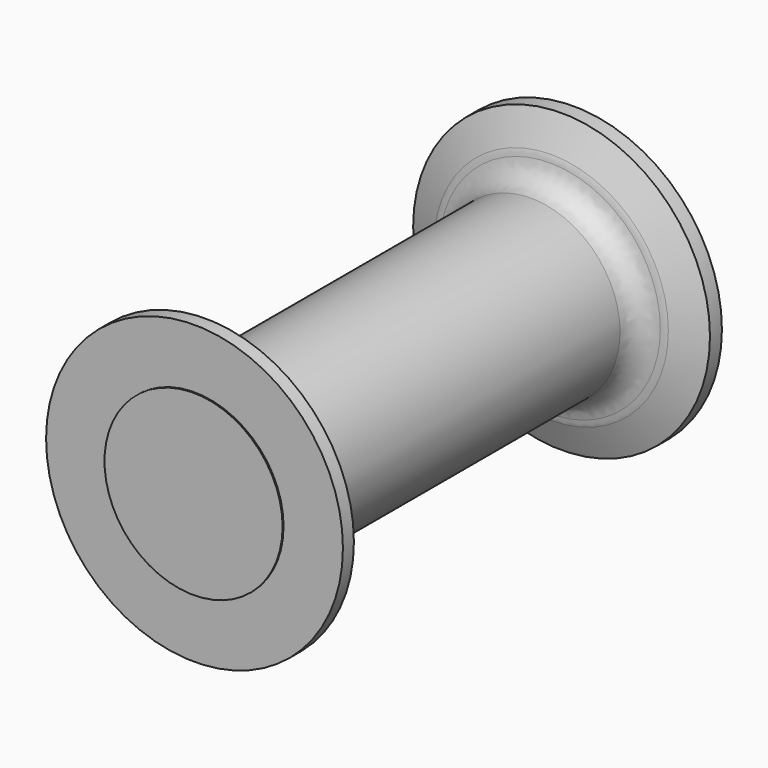
from build123d import *

# Parameters (mm, degrees)
F0_R     = 19.05
F1_DEPTH = 101.6
F2_R     = 31.75
F3_DEPTH = 6.35
F5_START = 95.25
F4_R     = 31.75
F5_DEPTH = 6.096
F6_SIZE  = 2.54
F8_R     = 5.08
F9_R     = 5.08


# Not quite as in the source:
# - a fillet or chamfer that OpenCascade refuses, or shapes differently, is made with other operations: its cross-section is extruded or revolved along the edge and cut away or added


with BuildPart() as f1:
    # F0 (on Front) → F1 (new body)
    with BuildSketch(Plane.XZ):
        Circle(F0_R)
    extrude(amount=F1_DEPTH)

    # F2 (on Front) → F3 (join)
    with BuildSketch(Plane.XZ):
        Circle(F2_R)
    extrude(amount=F3_DEPTH)

    # F4 (on Front) → F5 (join)
    with BuildSketch(Plane.XZ.offset(F5_START)):
        Circle(F4_R)
    extrude(amount=F5_DEPTH)

    # F6
    f6_edges = [f1.edges().sort_by_distance(p)[0] for p in [
        (-31.75, -6.35, 0),
        (-31.75, -95.25, 0),
    ]]
    chamfer(f6_edges, length=F6_SIZE)

    # F7: chamfer of 5.08 on 2 edges, made by hand

    # F7_s1 → F7_t2 (revolve, cut)
    with BuildSketch(Plane.XY):
        Polygon((24.13, -95.25), (32.8021024484, -98.8421024484), (29.21, -95.25), align=None)
    revolve(axis=Axis((0, -95.25, 0), (0, -1, 0)), mode=Mode.SUBTRACT)

    # F7_s3 → F7_t4 (revolve, cut)
    with BuildSketch(Plane.XY):
        Polygon((32.8021024484, -2.7578975516), (24.13, -6.35), (29.21, -6.35), align=None)
    revolve(axis=Axis((0, -6.35, 0), (0, -1, 0)), mode=Mode.SUBTRACT)

    # F8
    f8_edges = [f1.edges().sort_by_distance(p)[0] for p in [
        (-24.13, -6.35, 0),
        (-24.13, -95.25, 0),
    ]]
    fillet(f8_edges, radius=F8_R)

    # F9
    f9_edges = [f1.edges().sort_by_distance(p)[0] for p in [
        (-19.05, -95.25, 0),
        (-19.05, -6.35, 0),
    ]]
    fillet(f9_edges, radius=F9_R)


solid = f1.part
